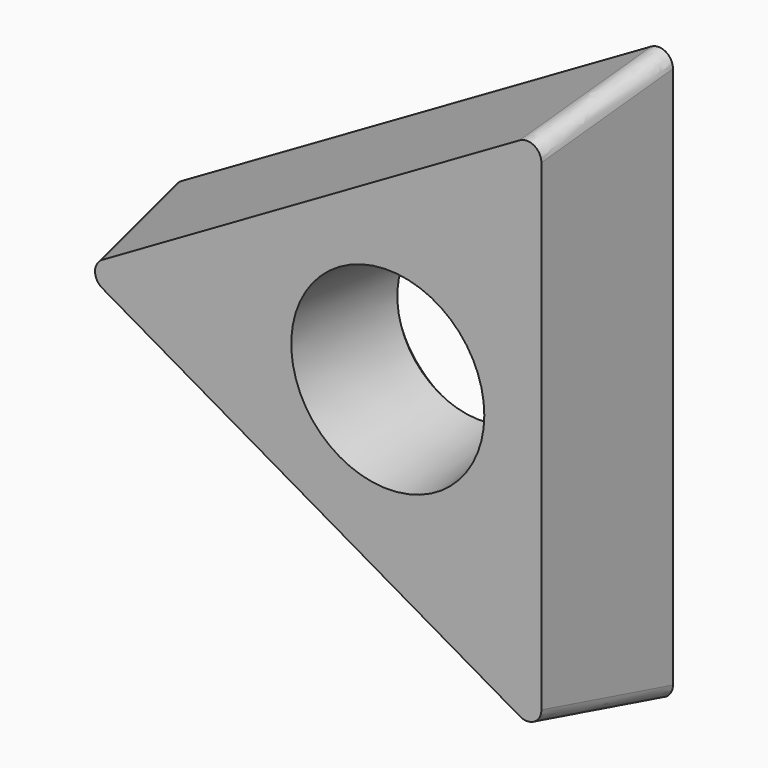
from build123d import *

# Parameters (mm, degrees)
F0_R     = 2.19964
F1_DEPTH = 3.97002
F1_TAPER = 7
F2_R     = 0.4064
F3_R     = 3.065431086
F4_DEPTH = 1.27
F4_TAPER = 45
F6_DEPTH = 0.2286
F6_TAPER = 50


# Not quite as in the source:
# - a feature names something its author has since deleted; it is built from what else it names


with BuildPart() as f1:
    # F0 (on Front) → F1 (new body)
    with BuildSketch(Plane.XZ):
        Polygon((4.7625, 8.248891971), (-9.525, 0), (4.7625, -8.248891971), align=None)
        Circle(F0_R, mode=Mode.SUBTRACT)
    extrude(amount=F1_DEPTH, taper=F1_TAPER)

    # F2
    f2_edges = [f1.edges().sort_by_distance(p)[0] for p in [
        (-9.037543, -1.98501, 0),
        (4.518771, -1.98501, 7.826742),
        (4.518771, -1.98501, -7.826742),
    ]]
    fillet(f2_edges, radius=F2_R)

    # F3 (on face) → F4 (cut)
    with BuildSketch(Plane.XZ):
        Circle(F3_R)
    extrude(amount=F4_DEPTH, taper=F4_TAPER, mode=Mode.SUBTRACT)

    # F5 (on face) → F6 (cut)
    with BuildSketch(Plane.XZ):
        with BuildLine():
            ThreePointArc((4.7625, 7.5449865229), (4.5593, 7.8969392469), (4.1529, 7.8969392469))
            Line((4.1529, 7.8969392469), (-8.9154, 0.3519527241))
            ThreePointArc((-8.9154, 0.3519527241), (-9.1186, 0), (-8.9154, -0.3519527241))
            Line((-8.9154, -0.3519527241), (4.1529, -7.8969392469))
            ThreePointArc((4.1529, -7.8969392469), (4.5593, -7.8969392469), (4.7625, -7.5449865229))
            Line((4.7625, -7.5449865229), (4.7625, 7.5449865229))
        make_face()
    extrude(amount=F6_DEPTH, taper=F6_TAPER, mode=Mode.SUBTRACT)


solid = f1.part
